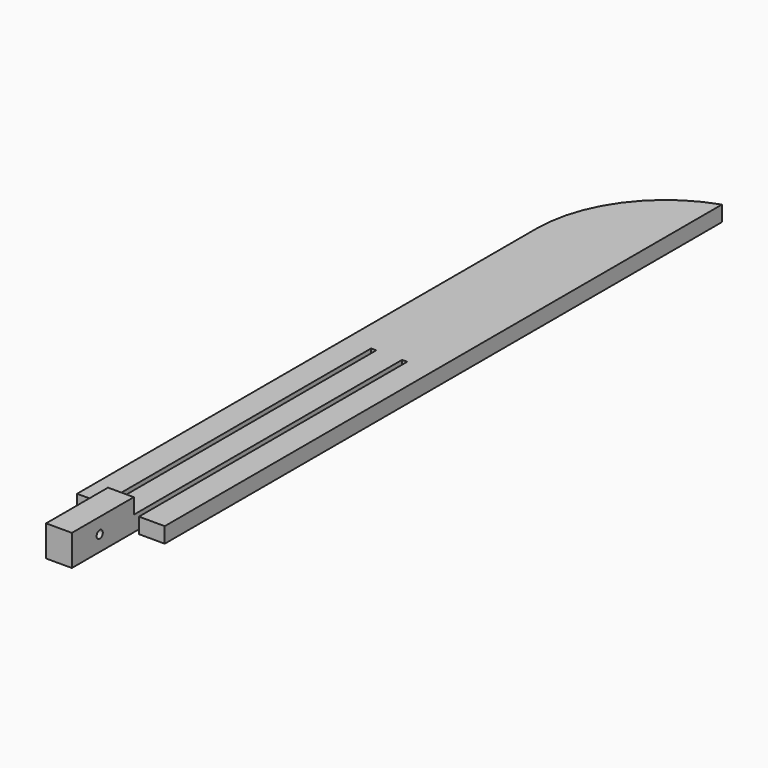
from build123d import *

# Parameters (mm, degrees)
F1_DEPTH    = 6
F2_T1_DEPTH = 242.8543856465
F3_W        = 10
F3_H        = 30
F4_DEPTH    = 6
F5_R        = 1.5
F6_DEPTH    = 10


# Not quite as in the source:
# - a fillet or chamfer that OpenCascade refuses, or shapes differently, is made with other operations: its cross-section is extruded or revolved along the edge and cut away or added


with BuildPart() as f1:
    # F0 (on Top) → F1 (new body)
    with BuildSketch(Plane.XY):
        Polygon((14.9102990106, 227.5062542017), (-19.0897009894, 227.5062542017), (-19.0897009894, -42.4937457983), (-9.0897009894, -42.4937457983), (-9.0897009894, 87.5062542017), (-7.0897009894, 87.5062542017), (-7.0897009894, -72.4937457983), (2.9102990106, -72.4937457983), (2.9102990106, 87.5062542017), (4.9102990106, 87.5062542017), (4.9102990106, -42.4937457983), (14.9102990106, -42.4937457983), align=None)
    extrude(amount=F1_DEPTH)

    # F2: fillet of radius 50 on 1 edges, made by hand

    # F2_s2 → F2_t1 (cut)
    with BuildSketch(Plane.XY.offset(-118.4271928233)):
        with BuildLine():
            ThreePointArc((14.9102990106, 227.5062542017), (-9.7098930126, 209.2901365467), (-19.0897009894, 180.1353770724))
            Line((-19.0897009894, 180.1353770724), (-19.0897009894, 227.5062542017))
            Line((-19.0897009894, 227.5062542017), (14.9102990106, 227.5062542017))
        make_face()
    extrude(amount=F2_T1_DEPTH, mode=Mode.SUBTRACT)

    # F3 (on face) → F4 (join)
    with BuildSketch(Plane.XY.offset(6)):
        with Locations((-2.0897009894, -57.4937457983)):
            Rectangle(F3_W, F3_H)
    extrude(amount=F4_DEPTH)

    # F5 (on face) → F6 (cut, through all)
    with BuildSketch(Plane(origin=(-7.0897009894, 0, 0), x_dir=(0, -1, 0), z_dir=(-1, 0, 0))):
        with Locations((59.0019002557, 6)):
            Circle(F5_R)
    extrude(amount=-F6_DEPTH, mode=Mode.SUBTRACT)


solid = f1.part
